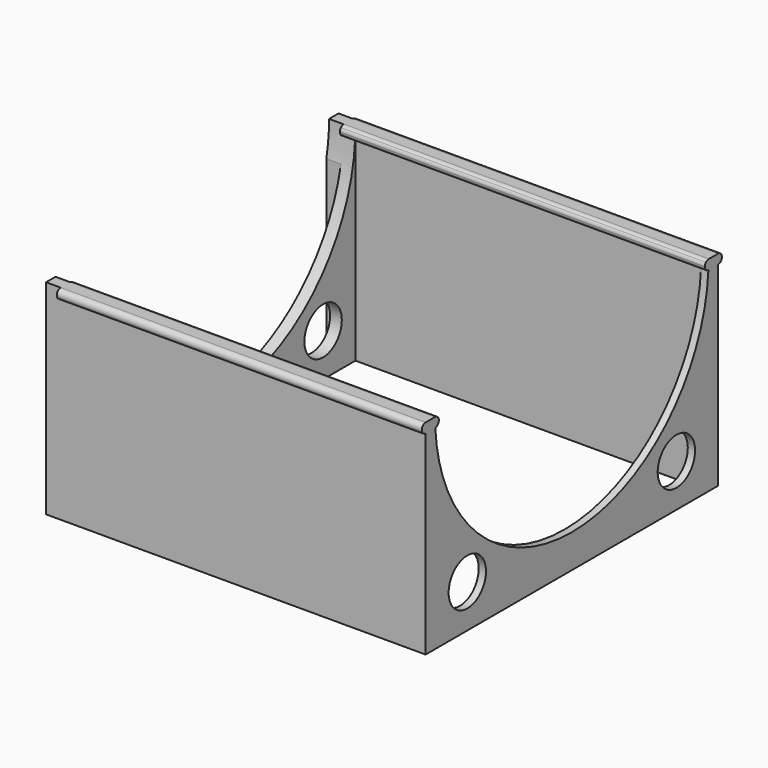
from build123d import *

# Parameters (mm, degrees)
F0_W     = 150.495
F0_H     = 148.844
F0_W_2   = 6.35
F0_H_2   = 6.604
F1_DEPTH = 88.9
F3_R     = 10.16
F4_DEPTH = 187.706
F2_R     = 2.0955
F5_DEPTH = 158.75


with BuildPart() as f1:
    # F0 (on Top) → F1 (new body)
    with BuildSketch(Plane.XY):
        Polygon((71.1090738666, 54.229), (-87.6409261334, 54.229), (-87.6409261334, 47.625), (-87.6409261334, 3.429), (-87.6409261334, -3.175), (-87.6409261334, -47.371), (-87.6409261334, -53.975), (-87.6409261334, -98.171), (-87.6409261334, -104.775), (71.1090738666, -104.775), align=None)
        with Locations((-7.3134261334, -25.273)):
            Rectangle(F0_W, F0_H, mode=Mode.SUBTRACT)
        with Locations((-90.8159261334, 50.927)):
            Rectangle(F0_W_2, F0_H_2)
        with Locations((-90.8159261334, 0.127)):
            Rectangle(F0_W_2, F0_H_2)
        with Locations((-90.8159261334, -50.673)):
            Rectangle(F0_W_2, F0_H_2)
        with Locations((-90.8159261334, -101.473)):
            Rectangle(F0_W_2, F0_H_2)
    extrude(amount=F1_DEPTH)

    # F3 (on face) → F4 (cut)
    with BuildSketch(Plane.YZ.offset(71.1090738666)):
        with BuildLine():
            ThreePointArc((-99.6304956393, 88.9), (-25.273, 14.5425043607), (49.0844956393, 88.9))
            Line((49.0844956393, 88.9), (-99.6304956393, 88.9))
        make_face()
        with Locations((-82.1161537051, 18.5863859951)):
            Circle(F3_R)
        with Locations((31.5701537051, 18.5863859951)):
            Circle(F3_R)
    extrude(amount=-F4_DEPTH, mode=Mode.SUBTRACT)

    # F2 (on face) → F5 (join, through all)
    with BuildSketch(Plane(origin=(-87.6409261334, 0, 0), x_dir=(0, -1, 0), z_dir=(-1, 0, 0))):
        with Locations((104.775, 86.8045)):
            Circle(F2_R)
        with Locations((-54.229, 86.8047326803)):
            Circle(F2_R)
        with BuildLine():
            ThreePointArc((-47.625, 85.3684040196), (-47.2016091494, 86.0328328215), (-47.0535, 86.8066474795))
            ThreePointArc((-47.0535, 86.8066474795), (-47.2016091494, 87.5804621376), (-47.625, 88.2448909395))
            Line((-47.625, 88.2448909395), (-47.625, 85.3684040196))
        make_face()
        with BuildLine():
            Line((-47.625, 85.3684040196), (-47.625, 88.2448909395))
            ThreePointArc((-47.625, 88.2448909395), (-51.2445, 86.8066474795), (-47.625, 85.3684040196))
        make_face()
        with Locations((99.695, 86.8045)):
            Circle(F2_R)
    extrude(amount=-F5_DEPTH)


solid = f1.part
